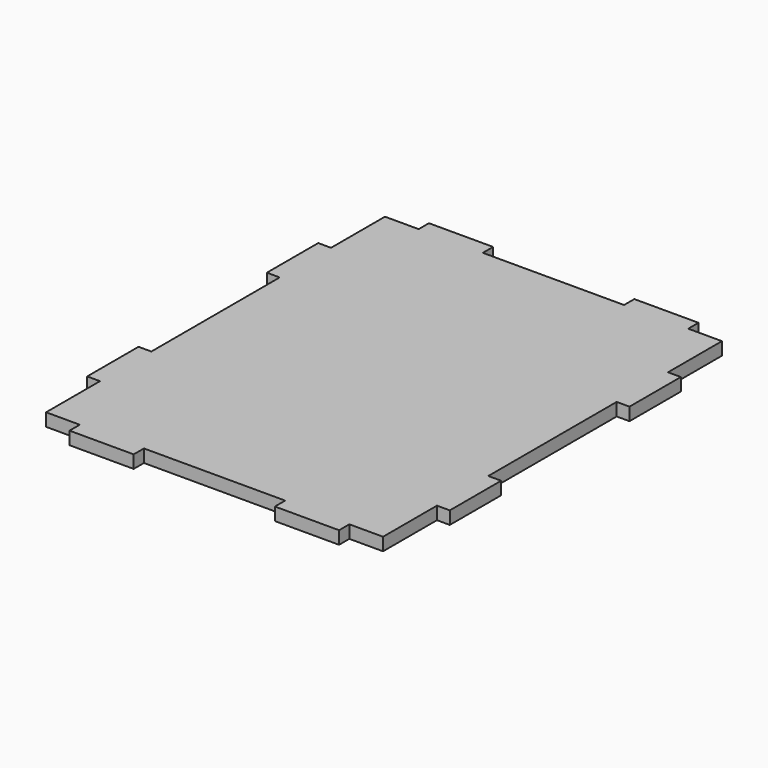
from build123d import *

# Parameters (mm, degrees)
F1_DEPTH = 4


# Not quite as in the source:
# - a feature names something its author has since deleted; it is built from what else it names


with BuildPart() as f1:
    # F0 (on Top) → F1 (new body)
    with BuildSketch(Plane.XY):
        Polygon((52.5, 45), (52.5, 66), (42, 66), (42, 70), (22, 70), (22, 66), (-22, 66), (-22, 70), (-42, 70), (-42, 66), (-52.5, 66), (-52.5, 45), (-56.5, 45), (-56.5, 25), (-52.5, 25), (-52.5, -25), (-56.5, -25), (-56.5, -45), (-52.5, -45), (-52.5, -66), (-42, -66), (-42, -70), (-22, -70), (-22, -66), (22, -66), (22, -70), (42, -70), (42, -66), (52.5, -66), (52.5, -45), (56.5, -45), (56.5, -25), (52.5, -25), (52.5, 25), (56.5, 25), (56.5, 45), align=None)
    extrude(amount=F1_DEPTH)


solid = f1.part
